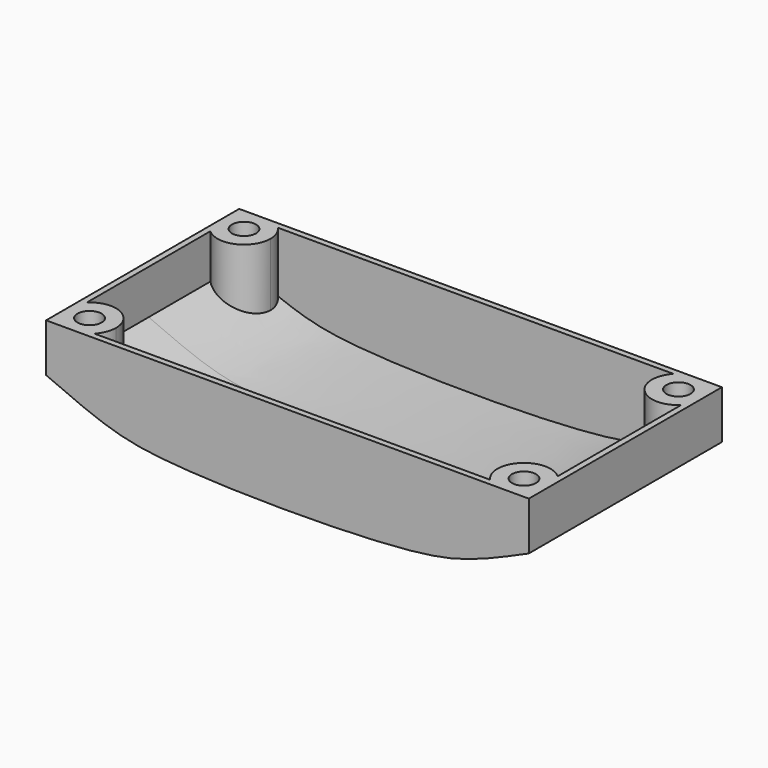
from build123d import *

# Parameters (mm, degrees)
F1_DEPTH = 50
F2_T     = -2.5
F3_R     = 5


with BuildPart() as f1:
    # F0 (on Front) → F1 (new body, symmetric)
    with BuildSketch(Plane.XZ):
        with BuildLine():
            Line((100, 20), (-100, 20))
            Line((-100, 20), (-100, 0))
            add(Edge.make_bspline(
                [(-100, 0), (-76.636724174, -10.24368871), (-58.0690404972, -17.3777106219), (57.5196598207, -17.5933090219), (77.717371285, -9.9781770259), (100, 0)],
                knots=[0, 0, 0, 0, 0.2955020731, 0.7044979269, 1, 1, 1, 1], degree=3))
            Line((100, 0), (100, 20))
        make_face()
    extrude(amount=F1_DEPTH, both=True)

    # F2
    f2_openings = [f1.faces().sort_by_distance(p)[0] for p in [
        (0, 0, 20),
    ]]
    offset(amount=F2_T, openings=f2_openings, kind=Kind.INTERSECTION)


with BuildPart() as f4:
    # F3 (on face) → F4 (new body, up to the next surface of F1)
    with BuildSketch(Plane.XY.offset(20)):
        with BuildLine():
            ThreePointArc((-81.9532615303, -47.5), (-79.7649102797, -44.0302528973), (-79, -40))
            ThreePointArc((-79, -40), (-85.6125178063, -29.9128794991), (-97.5, -31.9532615303))
            Line((-97.5, -31.9532615303), (-97.5, -47.5))
            Line((-97.5, -47.5), (-81.9532615303, -47.5))
        make_face()
        with Locations((-90, -40)):
            Circle(F3_R, mode=Mode.SUBTRACT)
    extrude(until=Until.NEXT, target=f1.part, dir=(0, 0, -1))


with BuildPart() as f5_1:
    # F5: instance of F4
    add(f4.part.mirror(Plane.XZ))


with BuildPart() as f1_1:
    add(f1.part)

    add(f4.part)  # F6 merges F4

    add(f5_1.part)  # F6 merges F5_1
    # F6: F4, F5_1 across plane
    add(f4.part.mirror(Plane.YZ))
    add(f5_1.part.mirror(Plane.YZ))


solid = f1_1.part
